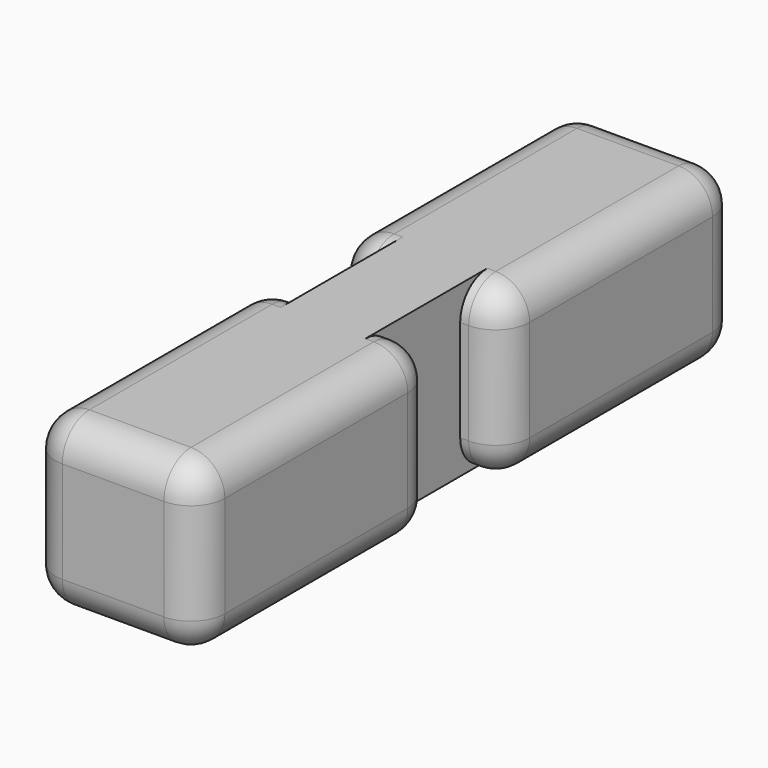
from build123d import *

# Parameters (mm, degrees)
F1_DEPTH     = 2
F2_R         = 0.4
F3_T1_DEPTH  = 2.7
F3_T3_DEPTH  = 2.7
F3_T5_DEPTH  = 0.1
F3_T7_DEPTH  = 0.1
F3_S11_W     = 0.4
F3_S11_H     = 0.4
F3_T12_DEPTH = 0.4
F3_S17_W     = 0.4
F3_S17_H     = 0.4
F3_T18_DEPTH = 0.4
F3_S23_W     = 0.4
F3_S23_H     = 0.4
F3_T24_DEPTH = 0.4
F3_S29_W     = 0.4
F3_S29_H     = 0.4
F3_T30_DEPTH = 0.4
F3_S35_W     = 0.4
F3_S35_H     = 0.4
F3_T36_DEPTH = 0.4
F3_S41_W     = 0.4
F3_S41_H     = 0.4
F3_T42_DEPTH = 0.4
F3_S47_W     = 0.4
F3_S47_H     = 0.4
F3_T48_DEPTH = 0.4
F3_S53_W     = 0.4
F3_S53_H     = 0.4
F3_T54_DEPTH = 0.4
F3_T58_ANGLE = 90
F3_T60_ANGLE = 90
F3_T62_ANGLE = 90
F3_T64_ANGLE = 90
F3_T66_ANGLE = 90
F3_T68_ANGLE = 90
F3_T70_ANGLE = 90
F3_T72_ANGLE = 90


# Not quite as in the source:
# - a fillet or chamfer that OpenCascade refuses, or shapes differently, is made with other operations: its cross-section is extruded or revolved along the edge and cut away or added


with BuildPart() as f1:
    # F0 (on Top) → F1 (new body)
    with BuildSketch(Plane.XY):
        Polygon((-1, -4), (1, -4), (1, -0.5), (0.5, -0.5), (0.5, 0.5), (1, 0.5), (1, 4), (-1, 4), (-1, 0.5), (-0.5, 0.5), (-0.5, -0.5), (-1, -0.5), align=None)
    extrude(amount=F1_DEPTH)

    # F2
    f2_edges = [f1.edges().sort_by_distance(p)[0] for p in [
        (0, -4, 2),
        (1, -4, 1),
        (-1, -4, 1),
        (0, -4, 0),
        (1, 4, 1),
        (0, 4, 2),
        (-1, 4, 1),
        (0, 4, 0),
        (1, 0.5, 1),
        (1, -0.5, 1),
        (-1, 0.5, 1),
        (-1, -0.5, 1),
    ]]
    fillet(f2_edges, radius=F2_R)

    # F3: fillet of radius 0.4 on 8 edges, made by hand

    # F3_s2 → F3_t1 (cut)
    with BuildSketch(Plane.XZ.offset(0.9)):
        with BuildLine():
            ThreePointArc((0.6, 2), (0.8828427125, 1.8828427125), (1, 1.6))
            Line((1, 1.6), (1, 2))
            Line((1, 2), (0.6, 2))
        make_face()
        with BuildLine():
            ThreePointArc((1, 0.4), (0.8828427125, 0.1171572875), (0.6, 0))
            Line((0.6, 0), (1, 0))
            Line((1, 0), (1, 0.4))
        make_face()
        with BuildLine():
            ThreePointArc((-0.6, 2), (-0.8828427125, 1.8828427125), (-1, 1.6))
            Line((-1, 1.6), (-1, 2))
            Line((-1, 2), (-0.6, 2))
        make_face()
        with BuildLine():
            ThreePointArc((-1, 0.4), (-0.8828427125, 0.1171572875), (-0.6, 0))
            Line((-0.6, 0), (-1, 0))
            Line((-1, 0), (-1, 0.4))
        make_face()
    extrude(amount=F3_T1_DEPTH, mode=Mode.SUBTRACT)

    # F3_s4 → F3_t3 (cut)
    with BuildSketch(Plane.XZ.offset(-3.6)):
        with BuildLine():
            ThreePointArc((0.6, 2), (0.8828427125, 1.8828427125), (1, 1.6))
            Line((1, 1.6), (1, 2))
            Line((1, 2), (0.6, 2))
        make_face()
        with BuildLine():
            ThreePointArc((0.6, 0), (0.8828427125, 0.1171572875), (1, 0.4))
            Line((1, 0.4), (1, 0))
            Line((1, 0), (0.6, 0))
        make_face()
        with BuildLine():
            ThreePointArc((-0.6, 2), (-0.8828427125, 1.8828427125), (-1, 1.6))
            Line((-1, 1.6), (-1, 2))
            Line((-1, 2), (-0.6, 2))
        make_face()
        with BuildLine():
            ThreePointArc((-0.6, 0), (-0.8828427125, 0.1171572875), (-1, 0.4))
            Line((-1, 0.4), (-1, 0))
            Line((-1, 0), (-0.6, 0))
        make_face()
    extrude(amount=F3_T3_DEPTH, mode=Mode.SUBTRACT)

    # F3_s6 → F3_t5 (cut)
    with BuildSketch(Plane.YZ.offset(-0.6)):
        with BuildLine():
            ThreePointArc((0.9, 0), (0.6171572875, 0.1171572875), (0.5, 0.4))
            Line((0.5, 0.4), (0.5, 0))
            Line((0.5, 0), (0.9, 0))
        make_face()
        with BuildLine():
            ThreePointArc((-0.9, 0), (-0.6171572875, 0.1171572875), (-0.5, 0.4))
            Line((-0.5, 0.4), (-0.5, 0))
            Line((-0.5, 0), (-0.9, 0))
        make_face()
        with BuildLine():
            ThreePointArc((0.9, 2), (0.6171572875, 1.8828427125), (0.5, 1.6))
            Line((0.5, 1.6), (0.5, 2))
            Line((0.5, 2), (0.9, 2))
        make_face()
        with BuildLine():
            ThreePointArc((-0.9, 2), (-0.6171572875, 1.8828427125), (-0.5, 1.6))
            Line((-0.5, 1.6), (-0.5, 2))
            Line((-0.5, 2), (-0.9, 2))
        make_face()
    extrude(amount=F3_T5_DEPTH, mode=Mode.SUBTRACT)

    # F3_s8 → F3_t7 (cut)
    with BuildSketch(Plane.YZ.offset(0.5)):
        with BuildLine():
            ThreePointArc((0.9, 0), (0.6171572875, 0.1171572875), (0.5, 0.4))
            Line((0.5, 0.4), (0.5, 0))
            Line((0.5, 0), (0.9, 0))
        make_face()
        with BuildLine():
            ThreePointArc((0.9, 2), (0.6171572875, 1.8828427125), (0.5, 1.6))
            Line((0.5, 1.6), (0.5, 2))
            Line((0.5, 2), (0.9, 2))
        make_face()
        with BuildLine():
            ThreePointArc((-0.9, 0), (-0.6171572875, 0.1171572875), (-0.5, 0.4))
            Line((-0.5, 0.4), (-0.5, 0))
            Line((-0.5, 0), (-0.9, 0))
        make_face()
        with BuildLine():
            ThreePointArc((-0.9, 2), (-0.6171572875, 1.8828427125), (-0.5, 1.6))
            Line((-0.5, 1.6), (-0.5, 2))
            Line((-0.5, 2), (-0.9, 2))
        make_face()
    extrude(amount=F3_T7_DEPTH, mode=Mode.SUBTRACT)


with BuildPart() as f3_tool10:
    # F3_s11 → F3_t12 (new body)
    with BuildSketch(Plane.XY.offset(0.4)):
        with Locations((-0.8, 3.8)):
            Rectangle(F3_S11_W, F3_S11_H)
    extrude(amount=-F3_T12_DEPTH)

    # F3_s13 → F3_t14 (revolve, cut)
    with BuildSketch(Plane(origin=(-0.6, 3.6, 0.4), x_dir=(0.7071067812, -0.7071067812, 0), z_dir=(0.7071067812, 0.7071067812, 0))):
        with BuildLine():
            ThreePointArc((0, -0.4), (0.4, 0), (0, 0.4))
            Line((0, 0.4), (0, -0.4))
        make_face()
    revolve(axis=Axis((-0.6, 3.6, 0.4), (0, 0, -1)), mode=Mode.SUBTRACT)


with BuildPart() as f1_1:
    add(f1.part)

    # F3_t9: cut F3_tool10
    add(f3_tool10.part, mode=Mode.SUBTRACT)


with BuildPart() as f3_tool16:
    # F3_s17 → F3_t18 (new body)
    with BuildSketch(Plane.YZ.offset(-0.6)):
        with Locations((-3.8, 0.2)):
            Rectangle(F3_S17_W, F3_S17_H)
    extrude(amount=-F3_T18_DEPTH)

    # F3_s19 → F3_t20 (revolve, cut)
    with BuildSketch(Plane(origin=(-0.6, -3.6, 0.4), x_dir=(0, 0.7071067812, 0.7071067812), z_dir=(0, -0.7071067812, 0.7071067812))):
        with BuildLine():
            ThreePointArc((0, -0.4), (0.4, 0), (0, 0.4))
            Line((0, 0.4), (0, -0.4))
        make_face()
    revolve(axis=Axis((-0.6, -3.6, 0.4), (-1, 0, 0)), mode=Mode.SUBTRACT)


with BuildPart() as f1_2:
    add(f1_1.part)

    # F3_t15: cut F3_tool16
    add(f3_tool16.part, mode=Mode.SUBTRACT)


with BuildPart() as f3_tool22:
    # F3_s23 → F3_t24 (new body)
    with BuildSketch(Plane.XY.offset(1.6)):
        with Locations((-0.8, 3.8)):
            Rectangle(F3_S23_W, F3_S23_H)
    extrude(amount=F3_T24_DEPTH)

    # F3_s25 → F3_t26 (revolve, cut)
    with BuildSketch(Plane(origin=(-0.6, 3.6, 1.6), x_dir=(0.7071067812, -0.7071067812, 0), z_dir=(-0.7071067812, -0.7071067812, 0))):
        with BuildLine():
            ThreePointArc((0, -0.4), (0.4, 0), (0, 0.4))
            Line((0, 0.4), (0, -0.4))
        make_face()
    revolve(axis=Axis((-0.6, 3.6, 1.6), (0, 0, 1)), mode=Mode.SUBTRACT)


with BuildPart() as f1_3:
    add(f1_2.part)

    # F3_t21: cut F3_tool22
    add(f3_tool22.part, mode=Mode.SUBTRACT)


with BuildPart() as f3_tool28:
    # F3_s29 → F3_t30 (new body)
    with BuildSketch(Plane.XY.offset(1.6)):
        with Locations((-0.8, -3.8)):
            Rectangle(F3_S29_W, F3_S29_H)
    extrude(amount=F3_T30_DEPTH)

    # F3_s31 → F3_t32 (revolve, cut)
    with BuildSketch(Plane(origin=(-0.6, -3.6, 1.6), x_dir=(0.7071067812, 0.7071067812, 0), z_dir=(0.7071067812, -0.7071067812, 0))):
        with BuildLine():
            ThreePointArc((0, -0.4), (0.4, 0), (0, 0.4))
            Line((0, 0.4), (0, -0.4))
        make_face()
    revolve(axis=Axis((-0.6, -3.6, 1.6), (0, 0, 1)), mode=Mode.SUBTRACT)


with BuildPart() as f1_4:
    add(f1_3.part)

    # F3_t27: cut F3_tool28
    add(f3_tool28.part, mode=Mode.SUBTRACT)


with BuildPart() as f3_tool34:
    # F3_s35 → F3_t36 (new body)
    with BuildSketch(Plane.XY.offset(0.4)):
        with Locations((0.8, 3.8)):
            Rectangle(F3_S35_W, F3_S35_H)
    extrude(amount=-F3_T36_DEPTH)

    # F3_s37 → F3_t38 (revolve, cut)
    with BuildSketch(Plane(origin=(0.6, 3.6, 0.4), x_dir=(-0.7071067812, -0.7071067812, 0), z_dir=(0.7071067812, -0.7071067812, 0))):
        with BuildLine():
            ThreePointArc((0, -0.4), (0.4, 0), (0, 0.4))
            Line((0, 0.4), (0, -0.4))
        make_face()
    revolve(axis=Axis((0.6, 3.6, 0.4), (0, 0, -1)), mode=Mode.SUBTRACT)


with BuildPart() as f1_5:
    add(f1_4.part)

    # F3_t33: cut F3_tool34
    add(f3_tool34.part, mode=Mode.SUBTRACT)


with BuildPart() as f3_tool40:
    # F3_s41 → F3_t42 (new body)
    with BuildSketch(Plane.XY.offset(1.6)):
        with Locations((0.8, 3.8)):
            Rectangle(F3_S41_W, F3_S41_H)
    extrude(amount=F3_T42_DEPTH)

    # F3_s43 → F3_t44 (revolve, cut)
    with BuildSketch(Plane(origin=(0.6, 3.6, 1.6), x_dir=(-0.7071067812, -0.7071067812, 0), z_dir=(-0.7071067812, 0.7071067812, 0))):
        with BuildLine():
            ThreePointArc((0, -0.4), (0.4, 0), (0, 0.4))
            Line((0, 0.4), (0, -0.4))
        make_face()
    revolve(axis=Axis((0.6, 3.6, 1.6), (0, 0, 1)), mode=Mode.SUBTRACT)


with BuildPart() as f1_6:
    add(f1_5.part)

    # F3_t39: cut F3_tool40
    add(f3_tool40.part, mode=Mode.SUBTRACT)


with BuildPart() as f3_tool46:
    # F3_s47 → F3_t48 (new body)
    with BuildSketch(Plane.YZ.offset(0.6)):
        with Locations((-3.8, 0.2)):
            Rectangle(F3_S47_W, F3_S47_H)
    extrude(amount=F3_T48_DEPTH)

    # F3_s49 → F3_t50 (revolve, cut)
    with BuildSketch(Plane(origin=(0.6, -3.6, 0.4), x_dir=(0, 0.7071067812, 0.7071067812), z_dir=(0, 0.7071067812, -0.7071067812))):
        with BuildLine():
            ThreePointArc((0, -0.4), (0.4, 0), (0, 0.4))
            Line((0, 0.4), (0, -0.4))
        make_face()
    revolve(axis=Axis((0.6, -3.6, 0.4), (1, 0, 0)), mode=Mode.SUBTRACT)


with BuildPart() as f1_7:
    add(f1_6.part)

    # F3_t45: cut F3_tool46
    add(f3_tool46.part, mode=Mode.SUBTRACT)


with BuildPart() as f3_tool52:
    # F3_s53 → F3_t54 (new body)
    with BuildSketch(Plane.XY.offset(1.6)):
        with Locations((0.8, -3.8)):
            Rectangle(F3_S53_W, F3_S53_H)
    extrude(amount=F3_T54_DEPTH)

    # F3_s55 → F3_t56 (revolve, cut)
    with BuildSketch(Plane(origin=(0.6, -3.6, 1.6), x_dir=(-0.7071067812, 0.7071067812, 0), z_dir=(0.7071067812, 0.7071067812, 0))):
        with BuildLine():
            ThreePointArc((0, -0.4), (0.4, 0), (0, 0.4))
            Line((0, 0.4), (0, -0.4))
        make_face()
    revolve(axis=Axis((0.6, -3.6, 1.6), (0, 0, 1)), mode=Mode.SUBTRACT)


with BuildPart() as f1_8:
    add(f1_7.part)

    # F3_t51: cut F3_tool52
    add(f3_tool52.part, mode=Mode.SUBTRACT)

    # F3_s57 → F3_t58 (revolve, cut)
    with BuildSketch(Plane.XZ.offset(-0.9)):
        with BuildLine():
            ThreePointArc((-0.6, 0), (-0.8828427125, 0.1171572875), (-1, 0.4))
            Line((-1, 0.4), (-1, 0))
            Line((-1, 0), (-0.6, 0))
        make_face()
    revolve(axis=Axis((-0.6, 0.9, 0), (0, 0, 1)), revolution_arc=F3_T58_ANGLE, mode=Mode.SUBTRACT)

    # F3_s59 → F3_t60 (revolve, cut)
    with BuildSketch(Plane.YZ.offset(-0.6)):
        with BuildLine():
            ThreePointArc((-0.9, 0), (-0.6171572875, 0.1171572875), (-0.5, 0.4))
            Line((-0.5, 0.4), (-0.5, 0))
            Line((-0.5, 0), (-0.9, 0))
        make_face()
    revolve(axis=Axis((-0.6, -0.9, 0), (0, 0, 1)), revolution_arc=F3_T60_ANGLE, mode=Mode.SUBTRACT)

    # F3_s61 → F3_t62 (revolve, cut)
    with BuildSketch(Plane.XZ.offset(-0.9)):
        with BuildLine():
            ThreePointArc((-0.6, 2), (-0.8828427125, 1.8828427125), (-1, 1.6))
            Line((-1, 1.6), (-1, 2))
            Line((-1, 2), (-0.6, 2))
        make_face()
    revolve(axis=Axis((-0.6, 0.9, 2), (0, 0, 1)), revolution_arc=F3_T62_ANGLE, mode=Mode.SUBTRACT)

    # F3_s63 → F3_t64 (revolve, cut)
    with BuildSketch(Plane.YZ.offset(-0.6)):
        with BuildLine():
            ThreePointArc((-0.9, 2), (-0.6171572875, 1.8828427125), (-0.5, 1.6))
            Line((-0.5, 1.6), (-0.5, 2))
            Line((-0.5, 2), (-0.9, 2))
        make_face()
    revolve(axis=Axis((-0.6, -0.9, 2), (0, 0, 1)), revolution_arc=F3_T64_ANGLE, mode=Mode.SUBTRACT)

    # F3_s65 → F3_t66 (revolve, cut)
    with BuildSketch(Plane.YZ.offset(0.6)):
        with BuildLine():
            ThreePointArc((0.9, 0), (0.6171572875, 0.1171572875), (0.5, 0.4))
            Line((0.5, 0.4), (0.5, 0))
            Line((0.5, 0), (0.9, 0))
        make_face()
    revolve(axis=Axis((0.6, 0.9, 0), (0, 0, 1)), revolution_arc=F3_T66_ANGLE, mode=Mode.SUBTRACT)

    # F3_s67 → F3_t68 (revolve, cut)
    with BuildSketch(Plane.YZ.offset(0.6)):
        with BuildLine():
            ThreePointArc((0.9, 2), (0.6171572875, 1.8828427125), (0.5, 1.6))
            Line((0.5, 1.6), (0.5, 2))
            Line((0.5, 2), (0.9, 2))
        make_face()
    revolve(axis=Axis((0.6, 0.9, 2), (0, 0, 1)), revolution_arc=F3_T68_ANGLE, mode=Mode.SUBTRACT)

    # F3_s69 → F3_t70 (revolve, cut)
    with BuildSketch(Plane.XZ.offset(0.9)):
        with BuildLine():
            ThreePointArc((0.6, 0), (0.8828427125, 0.1171572875), (1, 0.4))
            Line((1, 0.4), (1, 0))
            Line((1, 0), (0.6, 0))
        make_face()
    revolve(axis=Axis((0.6, -0.9, 0), (0, 0, 1)), revolution_arc=F3_T70_ANGLE, mode=Mode.SUBTRACT)

    # F3_s71 → F3_t72 (revolve, cut)
    with BuildSketch(Plane.XZ.offset(0.9)):
        with BuildLine():
            ThreePointArc((0.6, 2), (0.8828427125, 1.8828427125), (1, 1.6))
            Line((1, 1.6), (1, 2))
            Line((1, 2), (0.6, 2))
        make_face()
    revolve(axis=Axis((0.6, -0.9, 2), (0, 0, 1)), revolution_arc=F3_T72_ANGLE, mode=Mode.SUBTRACT)


solid = f1_8.part
